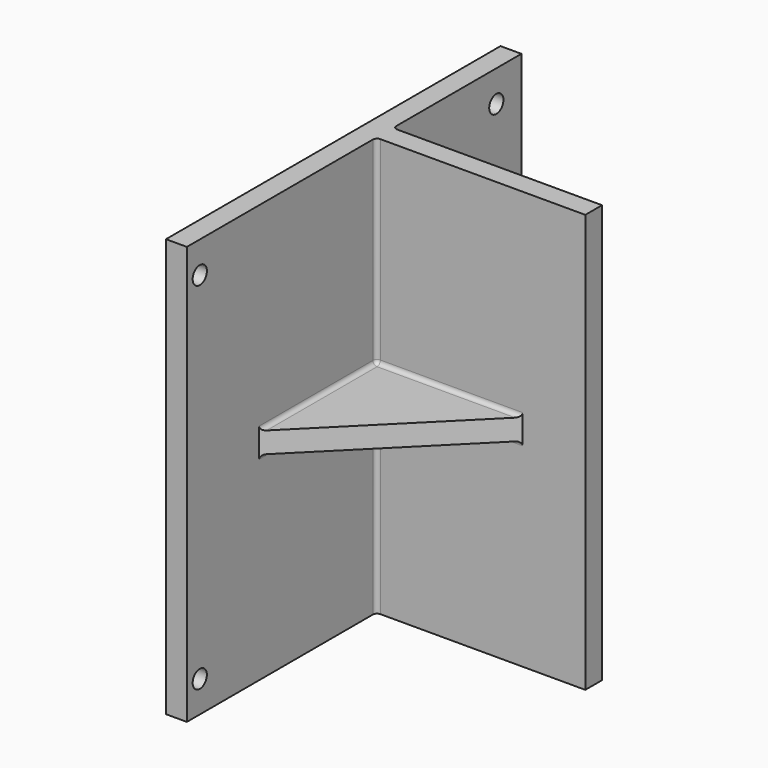
from build123d import *

# Parameters (mm, degrees)
F1_DEPTH     = 100
F2_W         = 70
F2_H         = 10
F3_DEPTH     = 100
F5_R         = 2
F6_DEPTH     = 25
F7_T1_DEPTH  = 200
F7_T6_DEPTH  = 73
F7_T11_DEPTH = 73
F7_T16_DEPTH = 73
F7_T21_DEPTH = 73
F7_T24_ANGLE = 90
F7_T26_ANGLE = 90
F9_D         = 8.5


# Not quite as in the source:
# - a fillet or chamfer that OpenCascade refuses, or shapes differently, is made with other operations: its cross-section is extruded or revolved along the edge and cut away or added


with BuildPart() as f1:
    # F0 (on Top) → F1 (new body, symmetric)
    with BuildSketch(Plane.XY):
        Polygon((10, 103.647416235), (0, 103.647416235), (0, -96.352583765), (10, -96.352583765), (10, 16.847416235), (110, 16.847416235), (110, 26.847416235), (10, 26.847416235), align=None)
    extrude(amount=F1_DEPTH, both=True)

    # F2 (on face) → F3 (join)
    with BuildSketch(Plane.YZ.offset(10)):
        with Locations((-18.152583765, 0)):
            Rectangle(F2_W, F2_H)
    extrude(amount=F3_DEPTH)

    # F5
    f5_edges = [f1.edges().sort_by_distance(p)[0] for p in [
        (10, 16.847416, 52.5),
        (10, 16.847416, -52.5),
    ]]
    fillet(f5_edges, radius=F5_R)

    # F4 (on face) → F6 (cut)
    with BuildSketch(Plane.XY.offset(5)):
        Polygon((110, -53.152583765), (110, 16.847416235), (80, 16.847416235), (10, -53.152583765), align=None)
    extrude(amount=-F6_DEPTH, mode=Mode.SUBTRACT)

    # F7: fillet of radius 2 on 5 edges, made by hand

    # F7_s2 → F7_t1 (join)
    with BuildSketch(Plane.XY.offset(-100)):
        with BuildLine():
            ThreePointArc((10, 28.847416235), (10.5857864376, 27.4332026726), (12, 26.847416235))
            Line((12, 26.847416235), (10, 26.847416235))
            Line((10, 26.847416235), (10, 28.847416235))
        make_face()
    extrude(amount=F7_T1_DEPTH)


with BuildPart() as f7_tool4:
    # F7_s5 → F7_t6 (new body)
    with BuildSketch(Plane.XZ.offset(-14.847416235)):
        with BuildLine():
            ThreePointArc((10, 7), (10.5857864376, 5.5857864376), (12, 5))
            Line((12, 5), (10, 5))
            Line((10, 5), (10, 7))
        make_face()
    extrude(amount=F7_T6_DEPTH)

    split(bisect_by=Plane(origin=(31.5762918825, -31.5762918825, 0), x_dir=(0, 0, 1), z_dir=(-0.7071067812, 0.7071067812, 0)), keep=Keep.TOP)


with BuildPart() as f1_1:
    add(f1.part)

    # F7_t3: union F7_tool4
    add(f7_tool4.part)


with BuildPart() as f7_tool9:
    # F7_s10 → F7_t11 (new body)
    with BuildSketch(Plane.YZ.offset(12)):
        with BuildLine():
            ThreePointArc((16.847416235, 7), (16.2616297973, 5.5857864376), (14.847416235, 5))
            Line((14.847416235, 5), (16.847416235, 5))
            Line((16.847416235, 5), (16.847416235, 7))
        make_face()
    extrude(amount=F7_T11_DEPTH)

    split(bisect_by=Plane(origin=(31.5762918825, -31.5762918825, 0), x_dir=(0, 0, 1), z_dir=(-0.7071067812, 0.7071067812, 0)), keep=Keep.TOP)


with BuildPart() as f1_2:
    add(f1_1.part)

    # F7_t8: union F7_tool9
    add(f7_tool9.part)


with BuildPart() as f7_tool14:
    # F7_s15 → F7_t16 (new body)
    with BuildSketch(Plane.XZ.offset(58.152583765)):
        with BuildLine():
            ThreePointArc((10, -7), (10.5857864376, -5.5857864376), (12, -5))
            Line((12, -5), (10, -5))
            Line((10, -5), (10, -7))
        make_face()
    extrude(amount=-F7_T16_DEPTH)

    split(bisect_by=Plane(origin=(31.5762918825, -31.5762918825, 0), x_dir=(0, 0, 1), z_dir=(-0.7071067812, 0.7071067812, 0)), keep=Keep.TOP)


with BuildPart() as f1_3:
    add(f1_2.part)

    # F7_t13: union F7_tool14
    add(f7_tool14.part)


with BuildPart() as f7_tool19:
    # F7_s20 → F7_t21 (new body)
    with BuildSketch(Plane.YZ.offset(12)):
        with BuildLine():
            ThreePointArc((16.847416235, -7), (16.2616297973, -5.5857864376), (14.847416235, -5))
            Line((14.847416235, -5), (16.847416235, -5))
            Line((16.847416235, -5), (16.847416235, -7))
        make_face()
    extrude(amount=F7_T21_DEPTH)

    split(bisect_by=Plane(origin=(31.5762918825, -31.5762918825, 0), x_dir=(0, 0, 1), z_dir=(-0.7071067812, 0.7071067812, 0)), keep=Keep.TOP)


with BuildPart() as f1_4:
    add(f1_3.part)

    # F7_t18: union F7_tool19
    add(f7_tool19.part)

    # F7_s23 → F7_t24 (revolve)
    with BuildSketch(Plane.YZ.offset(12)):
        with BuildLine():
            ThreePointArc((16.847416235, -7), (16.2616297973, -5.5857864376), (14.847416235, -5))
            Line((14.847416235, -5), (16.847416235, -5))
            Line((16.847416235, -5), (16.847416235, -7))
        make_face()
    revolve(axis=Axis((12, 14.847416235, -5), (0, 0, 1)), revolution_arc=F7_T24_ANGLE)

    # F7_s25 → F7_t26 (revolve)
    with BuildSketch(Plane.XZ.offset(-14.847416235)):
        with BuildLine():
            ThreePointArc((12, 5), (10.5857864376, 5.5857864376), (10, 7))
            Line((10, 7), (10, 5))
            Line((10, 5), (12, 5))
        make_face()
    revolve(axis=Axis((12, 14.847416235, 5), (0, 0, -1)), revolution_arc=F7_T26_ANGLE)

    # F9 (through all)
    with Locations(Plane.YZ.offset(10)):
        with Locations((88.647416235, 85), (88.647416235, -85), (-88.647416235, -85), (-88.647416235, 85)):
            Hole(F9_D / 2)


solid = f1_4.part
